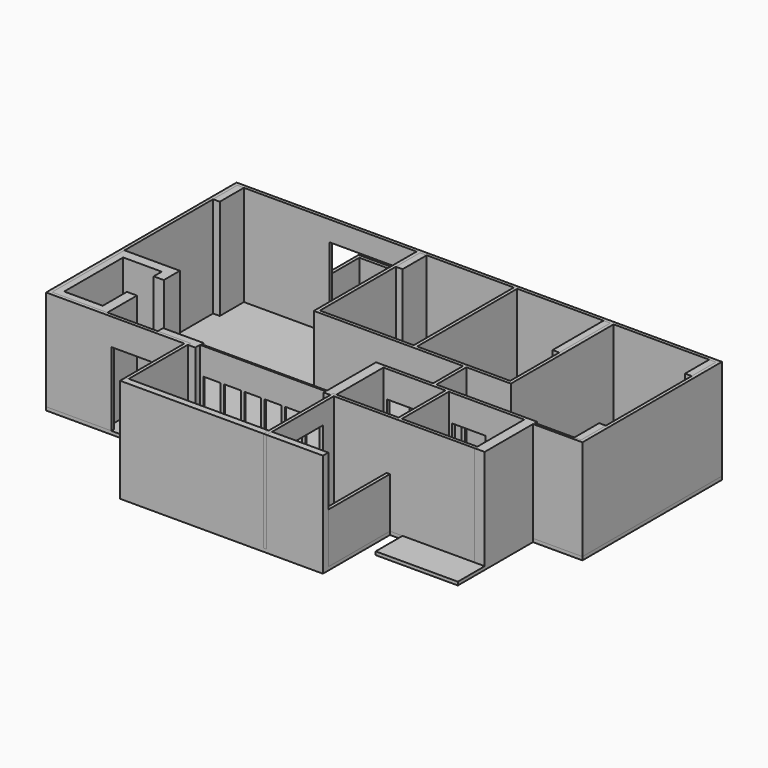
from build123d import *

# Parameters (mm, degrees)
F1_DEPTH  = 100
F3_DEPTH  = 3000
F4_W      = 300
F4_H      = 1000
F4_H_2    = 2000
F4_H_3    = 1950
F4_W_2    = 1200
F4_H_4    = 300
F4_W_3    = 6050
F4_H_5    = 200
F5_DEPTH  = 3000
F6_W      = 2750
F6_H      = 100
F7_DEPTH  = 3000
F8_W      = 2800
F8_H      = 3730
F8_W_2    = 2775
F9_DEPTH  = 3000
F10_W     = 1200
F10_H     = 2200
F11_DEPTH = 100
F12_W     = 1000
F12_H     = 2200
F13_DEPTH = 100
F14_W     = 1000
F14_H     = 2200
F15_DEPTH = 100
F16_W     = 1000
F16_H     = 2200
F17_DEPTH = 100
F18_W     = 1600
F18_H     = 2400
F19_DEPTH = 100
F20_W     = 2300
F20_H     = 2400
F21_DEPTH = 100
F22_W     = 100
F22_H     = 2300
F23_DEPTH = 1500
F24_W     = 3750
F24_H     = 50
F25_DEPTH = 3000
F26_W     = 510
F26_H     = 2000
F26_W_2   = 505
F27_DEPTH = 8100.001


with BuildPart() as f1:
    # F0 (on Top) → F1 (new body)
    with BuildSketch(Plane.XY):
        Polygon((-4125, 0), (0, 0), (0, -2400), (6050, -2400), (6050, -900), (6050, 0), (6050, 100), (6425, 100), (6425, 0), (6425, -900), (8875, -900), (8875, 1900), (10350, 1900), (10350, 7100), (1175, 7100), (1175, 8275), (-1425, 8275), (-1425, 7100), (-4125, 7100), align=None)
    extrude(amount=-F1_DEPTH)

    # F2 (on face) → F3 (join)
    with BuildSketch(Plane.XY):
        Polygon((-4125, 2800), (-4125, 0), (-2375, 0), (-2375, 1200), (-2675, 1200), (-2675, 300), (-3825, 300), (-3825, 2500), (-2675, 2500), (-2675, 2200), (-2375, 2200), (-2375, 2800), align=None)
    extrude(amount=F3_DEPTH)

    # F4 (on face) → F5 (join)
    with BuildSketch(Plane.XY):
        with Locations((-3975, 6600)):
            Rectangle(F4_W, F4_H)
        with Locations((1475, 6600)):
            Rectangle(F4_W, F4_H)
        with Locations((7050, 6100)):
            Rectangle(F4_W, F4_H_2)
        with Locations((10200, 6600)):
            Rectangle(F4_W, F4_H)
        with Locations((10200, 2400)):
            Rectangle(F4_W, F4_H)
        with Locations((8725, 1075)):
            Rectangle(F4_W, F4_H_3)
        with Locations((4225, 1075)):
            Rectangle(F4_W, F4_H_3)
        with Locations((-275, 150)):
            Rectangle(F4_W_2, F4_H_4)
        with Locations((3025, -2300)):
            Rectangle(F4_W_3, F4_H_5)
    extrude(amount=F5_DEPTH)


with BuildPart() as f7:
    # F6 (on face) → F7 (new body)
    with BuildSketch(Plane.XY):
        Polygon((0, 0), (0, -2200), (100, -2200), (100, 100), (-4025, 100), (-4025, 7000), (-1425, 7000), (-1425, 7100), (-4125, 7100), (-4125, 0), align=None)
        with Locations((-50, 7050)):
            Rectangle(F6_W, F6_H)
    extrude(amount=F7_DEPTH)

    # F8 (on face) → F9 (join)
    with BuildSketch(Plane.XY):
        Polygon((5875, 3170), (7200, 3170), (7200, 7000), (7200, 7100), (1325, 7100), (1325, 3170), (5775, 3170), (5775, 2050), (4375, 2050), (4375, 1950), (6225, 1950), (6225, 200), (4375, 200), (4375, 100), (8575, 100), (8575, 200), (6325, 200), (6325, 1950), (8575, 1950), (8575, 2050), (5875, 2050), align=None)
        with Locations((2825, 5135)):
            Rectangle(F8_W, F8_H, mode=Mode.SUBTRACT)
        with Locations((5712.5, 5135)):
            Rectangle(F8_W_2, F8_H, mode=Mode.SUBTRACT)
        Polygon((7200, 7100), (7200, 7000), (10250, 7000), (10250, 1975), (8875, 1975), (8875, 1900), (10250, 1900), (10350, 1900), (10350, 7000), (10350, 7100), (10250, 7100), align=None)
        Polygon((4375, -2400), (4375, 100), (4375, 200), (4275, 200), (4275, -2400), align=None)
    extrude(amount=F9_DEPTH)

    # F10 (on face) → F11 (cut)
    with BuildSketch(Plane.XZ):
        with Locations((-1575, 1100)):
            Rectangle(F10_W, F10_H)
    extrude(amount=-F11_DEPTH, mode=Mode.SUBTRACT)

    # F12 (on face) → F13 (cut)
    with BuildSketch(Plane.XZ.offset(-3170)):
        with Locations((3675, 1100)):
            Rectangle(F12_W, F12_H)
        with Locations((4975, 1100)):
            Rectangle(F12_W, F12_H)
    extrude(amount=-F13_DEPTH, mode=Mode.SUBTRACT)

    # F14 (on face) → F15 (cut)
    with BuildSketch(Plane(origin=(5775, 0, 0), x_dir=(0, -1, 0), z_dir=(-1, 0, 0))):
        with Locations((-2610, 1100)):
            Rectangle(F14_W, F14_H)
    extrude(amount=-F15_DEPTH, mode=Mode.SUBTRACT)

    # F16 (on face) → F17 (cut)
    with BuildSketch(Plane(origin=(0, 2050, 0), x_dir=(-1, 0, 0), z_dir=(0, 1, 0))):
        with Locations((-4975, 1100)):
            Rectangle(F16_W, F16_H)
        with Locations((-6925, 1100)):
            Rectangle(F16_W, F16_H)
    extrude(amount=-F17_DEPTH, mode=Mode.SUBTRACT)

    # F18 (on face) → F19 (cut)
    with BuildSketch(Plane(origin=(4275, 0, 0), x_dir=(0, -1, 0), z_dir=(-1, 0, 0))):
        with Locations((1100, 1200)):
            Rectangle(F18_W, F18_H)
    extrude(amount=-F19_DEPTH, mode=Mode.SUBTRACT)

    # F20 (on face) → F21 (cut)
    with BuildSketch(Plane.XZ.offset(-7000)):
        with Locations((-125, 1200)):
            Rectangle(F20_W, F20_H)
    extrude(amount=-F21_DEPTH, mode=Mode.SUBTRACT)

    # F22 (on face) → F23 (join)
    with BuildSketch(Plane.XY):
        Polygon((-1425, 8275), (-1425, 7100), (-1325, 7100), (-1325, 8175), (1075, 8175), (1075, 7100), (1175, 7100), (1175, 8275), align=None)
        with Locations((6000, -1050)):
            Rectangle(F22_W, F22_H)
    extrude(amount=F23_DEPTH)


with BuildPart() as f25:
    # F24 (on face) → F25 (new body)
    with BuildSketch(Plane.XY):
        with Locations((2200, 200)):
            Rectangle(F24_W, F24_H)
    extrude(amount=F25_DEPTH)

    # F26 (on face) → F27 (cut, through all)
    with BuildSketch(Plane.XZ.offset(-175)):
        with Locations((680, 1200)):
            Rectangle(F26_W, F26_H)
        with Locations((1290, 1200)):
            Rectangle(F26_W, F26_H)
        with Locations((1897.5, 1200)):
            Rectangle(F26_W_2, F26_H)
        with Locations((3720, 1200)):
            Rectangle(F26_W, F26_H)
        with Locations((2502.5, 1200)):
            Rectangle(F26_W_2, F26_H)
        with Locations((3110, 1200)):
            Rectangle(F26_W, F26_H)
    extrude(amount=-F27_DEPTH, mode=Mode.SUBTRACT)


solid = Compound([f1.part, f7.part, f25.part])
